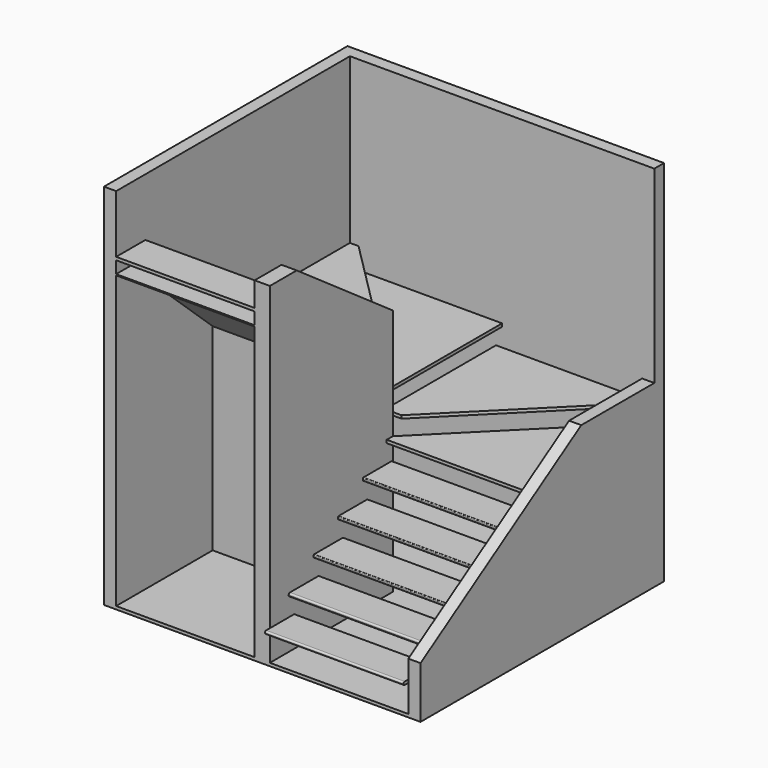
from build123d import *

# Parameters (mm, degrees)
F2_DEPTH  = 3048
F4_W      = 1155.7
F4_H      = 304.8
F5_DEPTH  = 25.4
F6_R      = 12.69999
F8_DEPTH  = 1155.7
F11_DEPTH = 25.4
F14_DEPTH = 25.4
F17_DEPTH = 25.4
F20_DEPTH = 25.4
F21_W     = 304.8
F21_H     = 25.4
F22_DEPTH = 1155.7
F24_W     = 2641.6
F24_H     = 2540
F25_DEPTH = 25.4
F23_W     = 127
F23_H     = 1282.7
F26_DEPTH = 2768.6
F28_DEPTH = 101.601
F30_DEPTH = 152.4
F32_DEPTH = 1155.7


# Not quite as in the source:
# - a fillet or chamfer is up to 0.001 mm smaller than in the source, because OpenCascade refuses the exact size


with BuildPart() as f2:
    # F1 (on Top) → F2 (new body)
    with BuildSketch(Plane.XY):
        Polygon((-1320.8, 0), (-1219.2, 0), (-1219.2, 2438.4), (1219.2, 2438.4), (1219.2, 0), (1320.8, 0), (1320.8, 2540), (-1320.8, 2540), align=None)
    extrude(amount=F2_DEPTH)

    # F4 (on offset) → F5 (join)
    with BuildSketch(Plane.XY.offset(254)):
        with Locations((641.35, 101.6)):
            Rectangle(F4_W, F4_H)
    extrude(amount=-F5_DEPTH)

    # F6 (radius 12.7 in the source; OpenCascade refuses exactly that, so slightly less here)
    f6_edges = [f2.edges().sort_by_distance(p)[0] for p in [
        (641.35, -50.8, 254),
        (641.35, -50.8, 228.6),
    ]]
    fillet(f6_edges, radius=F6_R)

    # F7 (on face) → F8 (join, through all)
    with BuildSketch(Plane(origin=(1219.2, 0, 0), x_dir=(0, -1, 0), z_dir=(-1, 0, 0))):
        with BuildLine():
            Line((-717.55, 787.4), (-1016, 787.4))
            Line((-1016, 787.4), (-1016, 762))
            Line((-1016, 762), (-717.55, 762))
            ThreePointArc((-717.55, 762), (-713.0598719395, 763.8598719395), (-711.2, 768.35))
            Line((-711.2, 768.35), (-711.2, 781.05))
            ThreePointArc((-711.2, 781.05), (-713.0598719395, 785.5401280605), (-717.55, 787.4))
        make_face()
        with BuildLine():
            Line((-463.55, 609.6), (-762, 609.6))
            Line((-762, 609.6), (-762, 584.2))
            Line((-762, 584.2), (-463.55, 584.2))
            ThreePointArc((-463.55, 584.2), (-459.0598719395, 586.0598719395), (-457.2, 590.55))
            Line((-457.2, 590.55), (-457.2, 603.25))
            ThreePointArc((-457.2, 603.25), (-459.0598719395, 607.7401280605), (-463.55, 609.6))
        make_face()
        with BuildLine():
            Line((-209.55, 431.8), (-508, 431.8))
            Line((-508, 431.8), (-508, 406.4))
            Line((-508, 406.4), (-203.2, 406.4))
            ThreePointArc((-203.2, 406.4), (-198.7098719395, 408.2598719395), (-196.85, 412.75))
            Line((-196.85, 412.75), (-196.85, 419.1))
            ThreePointArc((-196.85, 419.1), (-200.5697438789, 428.0802561211), (-209.55, 431.8))
        make_face()
        with BuildLine():
            Line((-1270, 939.8), (-977.9, 939.8))
            ThreePointArc((-977.9, 939.8), (-973.4098719395, 941.6598719395), (-971.55, 946.15))
            Line((-971.55, 946.15), (-971.55, 958.85))
            ThreePointArc((-971.55, 958.85), (-973.4098719395, 963.3401280605), (-977.9, 965.2))
            Line((-977.9, 965.2), (-1270, 965.2))
            Line((-1270, 965.2), (-1270, 939.8))
        make_face()
    extrude(amount=F8_DEPTH)

    # F10 (on offset) → F11 (join)
    with BuildSketch(Plane.XY.offset(1143)):
        Polygon((1219.2, 2438.4), (63.5, 1282.7), (63.5, 1219.2), (1219.2, 1219.2), align=None)
    extrude(amount=-F11_DEPTH)

    # F13 (on offset) → F14 (join)
    with BuildSketch(Plane.XY.offset(1320.8)):
        Polygon((0, 2438.4), (0, 1282.7), (135.3420489686, 1282.7), (1219.2, 2366.5579510314), (1219.2, 2438.4), align=None)
    extrude(amount=-F14_DEPTH)

    # F16 (on offset) → F17 (join)
    with BuildSketch(Plane.XY.offset(1498.6)):
        Polygon((-1219.2, 2438.4), (-63.5, 1282.7), (50.8, 1282.7), (50.8, 2438.4), align=None)
    extrude(amount=-F17_DEPTH)

    # F19 (on offset) → F20 (join)
    with BuildSketch(Plane.XY.offset(1676.4)):
        Polygon((-1219.2, 2438.4), (-1219.2, 1270), (-63.5, 1270), (-63.5, 1354.5420489686), (-1147.3579510314, 2438.4), align=None)
    extrude(amount=-F20_DEPTH)

    # F21 (on face) → F22 (join)
    with BuildSketch(Plane.YZ.offset(-1219.2)):
        with Locations((1168.4, 1841.5)):
            Rectangle(F21_W, F21_H)
        with Locations((914.4, 2019.3)):
            Rectangle(F21_W, F21_H)
        with Locations((660.4, 2197.1)):
            Rectangle(F21_W, F21_H)
        with Locations((406.4, 2374.9)):
            Rectangle(F21_W, F21_H)
        with Locations((152.4, 2552.7)):
            Rectangle(F21_W, F21_H)
    extrude(amount=F22_DEPTH)

    # F24 (on face) → F25 (join)
    with BuildSketch(Plane(origin=(0, 0, 0), x_dir=(1, 0, 0), z_dir=(0, 0, -1))):
        with Locations((0, -1270)):
            Rectangle(F24_W, F24_H)
    extrude(amount=F25_DEPTH)

    # F23 (on Top) → F26 (join)
    with BuildSketch(Plane.XY):
        with Locations((0, 641.35)):
            Rectangle(F23_W, F23_H)
    extrude(amount=F26_DEPTH)

    # F27 (on face) → F28 (cut, through all)
    with BuildSketch(Plane(origin=(1219.2, 0, 0), x_dir=(0, -1, 0), z_dir=(-1, 0, 0))):
        Polygon((-1676.4, 1473.2), (0, 406.4), (0, 3048), (-2438.4, 3048), (-2438.4, 1473.2), align=None)
    extrude(amount=-F28_DEPTH, mode=Mode.SUBTRACT)

    # F29 (on face) → F30 (cut)
    with BuildSketch(Plane.YZ.offset(63.5)):
        Polygon((1282.7, 2768.6), (280.2684394054, 2768.6), (1282.7, 2066.8979075838), align=None)
    extrude(amount=-F30_DEPTH, mode=Mode.SUBTRACT)

    # F31 (on face) → F32 (join, through all)
    with BuildSketch(Plane(origin=(-63.5, 0, 0), x_dir=(0, -1, 0), z_dir=(-1, 0, 0))):
        Polygon((-152.4, 2438.4), (-1016, 1651), (-1016, 0), (-1006.475, 0), (-1006.475, 1646.7947494006), (-148.7095638587, 2428.875), (0, 2428.875), (0, 2438.4), align=None)
    extrude(amount=F32_DEPTH)


solid = f2.part
